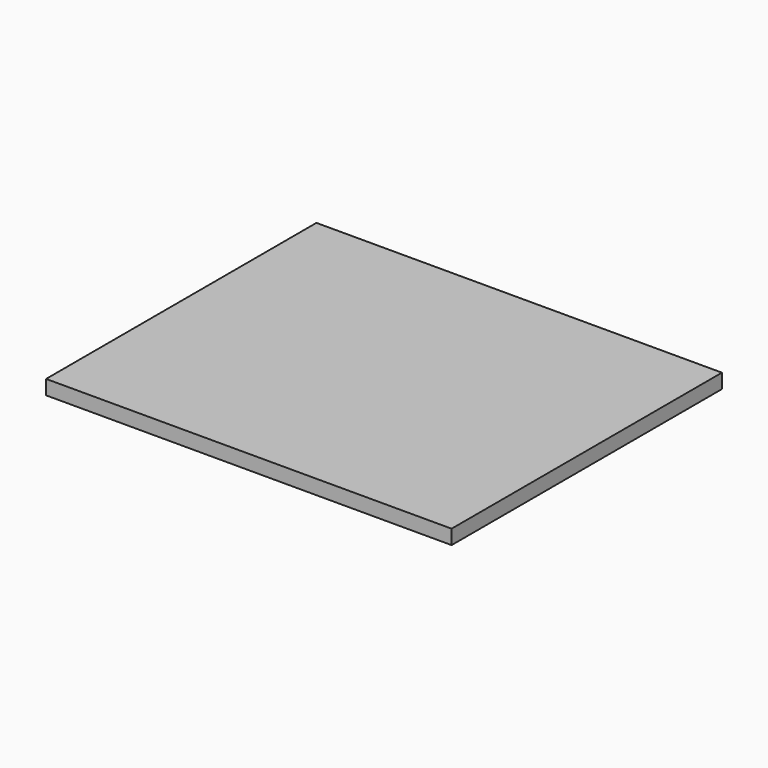
from build123d import *

# Parameters (mm, degrees)
F1_DEPTH = 70
F3_DEPTH = 2


# Not quite as in the source:
# - a feature names something its author has since deleted; it is built from what else it names


with BuildPart() as f1:
    # F0 (on Front) → F1 (new body)
    with BuildSketch(Plane.XZ):
        Polygon((0, -20), (0, -23), (32, -23), (32, -21), (38, -21), (42, -21), (42, -20), align=None)
        Polygon((-32, -23), (0, -23), (0, -20), (-17, -20), (-21, -20), (-30, -20), (-34, -20), (-34, -21), (-32, -21), align=None)
        Polygon((32, -21), (32, -23), (38, -23), (38, -22.25), (38, -21), align=None)
        Polygon((-38, -23), (-32, -23), (-32, -21), (-34, -21), (-38, -21), (-38, -22.25), align=None)
        Polygon((38, -22.25), (38, -23), (42, -23), (42, -21), (38, -21), align=None)
        Polygon((-42, -23), (-38, -23), (-38, -22.25), (-38, -21), (-42, -21), align=None)
        Polygon((-38, -21), (-34, -21), (-34, -20), (-42, -20), (-42, -21), align=None)
    extrude(amount=F1_DEPTH)

    # F2 (on face) → F3 (cut)
    with BuildSketch(Plane(origin=(0, 0, -23), x_dir=(1, 0, 0), z_dir=(0, 0, -1))):
        Polygon((-32, 28), (-42, 13.7185199326), (-42, 7), (-32, 21.2814800674), align=None)
        Polygon((-32, 63), (-42, 48.7185199326), (-42, 42), (-32, 56.2814800674), align=None)
    extrude(amount=-F3_DEPTH, mode=Mode.SUBTRACT)


solid = f1.part
